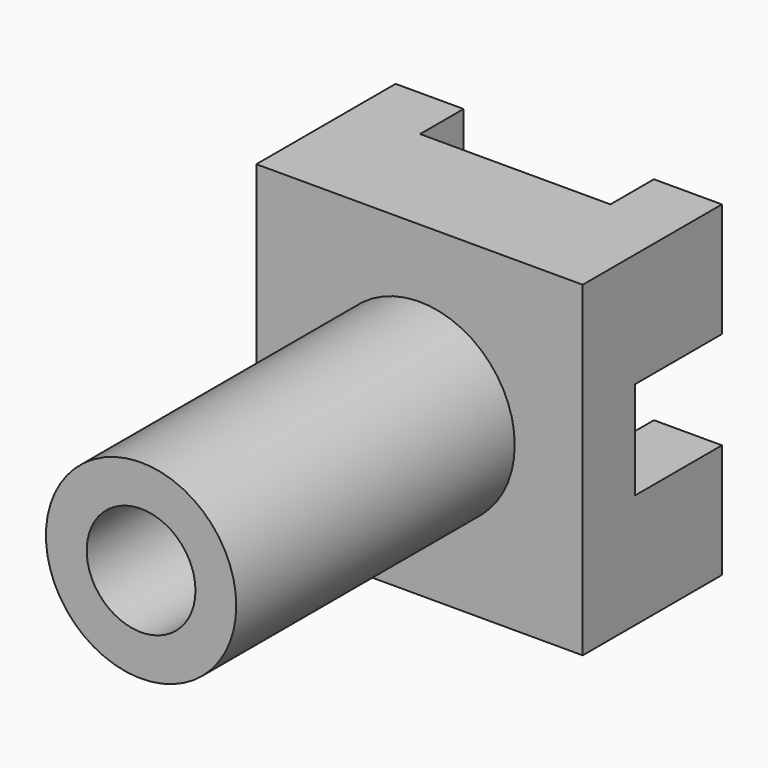
from build123d import *

# Parameters (mm, degrees)
F0_R     = 17.5
F0_R_2   = 10
F1_DEPTH = 64
F2_W     = 60
F2_H     = 60
F2_R     = 17.5
F2_R_2   = 10
F3_DEPTH = 32
F4_W     = 35
F4_H     = 10
F5_DEPTH = 60.001
F6_W     = 20
F6_H     = 18
F7_DEPTH = 60.001


with BuildPart() as f1:
    # F0 (on Front) → F1 (new body)
    with BuildSketch(Plane.XZ):
        Circle(F0_R)
        Circle(F0_R_2, mode=Mode.SUBTRACT)
    extrude(amount=F1_DEPTH)

    # F2 (on face) → F3 (join)
    with BuildSketch(Plane(origin=(0, 0, 0), x_dir=(-1, 0, 0), z_dir=(0, 1, 0))):
        Rectangle(F2_W, F2_H)
        Circle(F2_R, mode=Mode.SUBTRACT)
        Circle(F2_R)
        Circle(F2_R_2, mode=Mode.SUBTRACT)
    extrude(amount=F3_DEPTH)

    # F4 (on face) → F5 (cut, through all)
    with BuildSketch(Plane(origin=(0, 0, -30), x_dir=(1, 0, 0), z_dir=(0, 0, -1))):
        with Locations((0, -27)):
            Rectangle(F4_W, F4_H)
    extrude(amount=-F5_DEPTH, mode=Mode.SUBTRACT)

    # F6 (on face) → F7 (cut, through all)
    with BuildSketch(Plane(origin=(-30, 0, 0), x_dir=(0, -1, 0), z_dir=(-1, 0, 0))):
        with Locations((-22, 0)):
            Rectangle(F6_W, F6_H)
    extrude(amount=-F7_DEPTH, mode=Mode.SUBTRACT)


solid = f1.part
